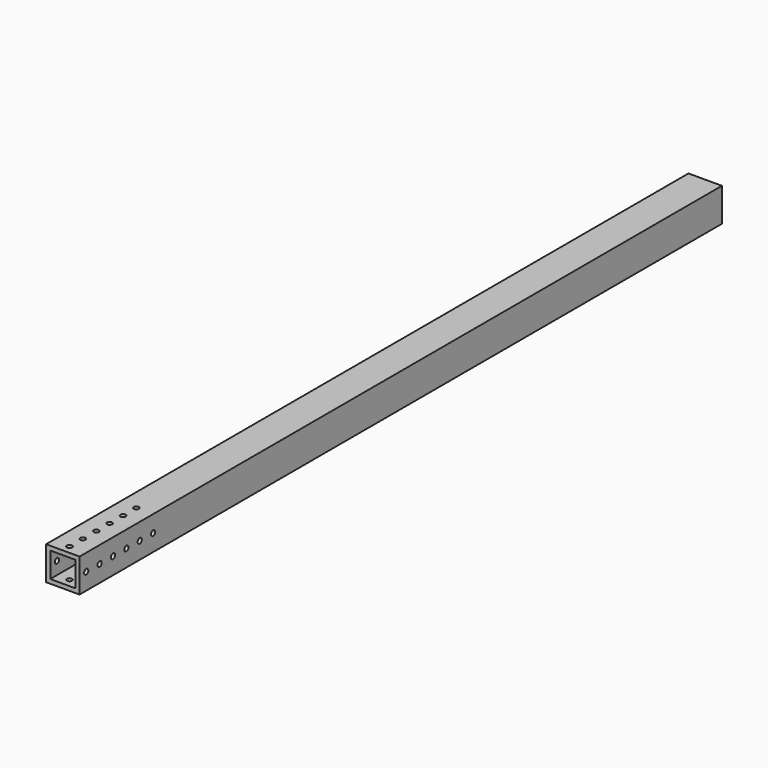
from build123d import *

# Parameters (mm, degrees)
F0_W     = 25.4
F0_H     = 25.4
F0_W_2   = 19.05
F0_H_2   = 19.05
F1_DEPTH = 304.8
F3_D     = 3.96875


# Not quite as in the source:
# - a pattern or mirror of a feature is missing from the dataset's text; its kind, count and spacing are read off the source's solid


with BuildPart() as f1:
    # F0 (on Front) → F1 (new body, symmetric)
    with BuildSketch(Plane.XZ):
        Rectangle(F0_W, F0_H)
        Rectangle(F0_W_2, F0_H_2, mode=Mode.SUBTRACT)
    extrude(amount=F1_DEPTH, both=True)

    # F3 (through all)
    with Locations(Plane.XY.offset(12.7)):
        with Locations((0, -234.95), (0, -247.65), (0, -260.35), (0, -273.05), (0, -285.75), (0, -298.45)):
            f3 = Hole(F3_D / 2)

    # F3_copies: F3 across plane
    add(f3.mirror(Plane(origin=(0, 0, 0), x_dir=(-0.7071067812, 0, -0.7071067812), z_dir=(0.7071067812, 0, -0.7071067812))), mode=Mode.SUBTRACT)


solid = f1.part
